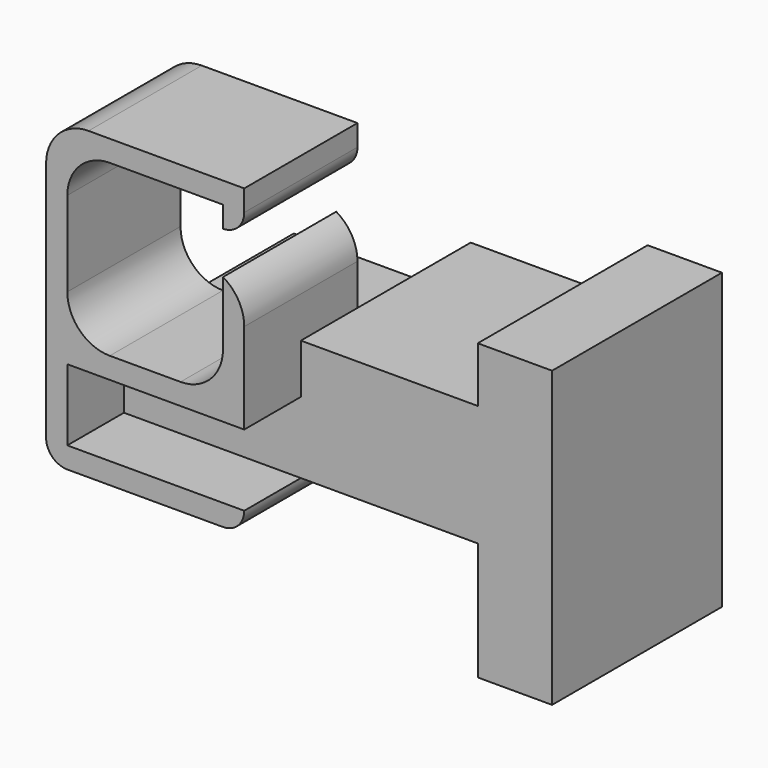
from build123d import *

# Parameters (mm, degrees)
F0_W          = 25
F0_H          = 7
F0_W_2        = 10.5
F0_H_2        = 10.1
F0_H_3        = 16.6735936701
F0_H_4        = 7.8
F1_DEPTH      = 15
F1_DEPTH_BACK = 15
F2_W          = 3
F2_H          = 3
F3_DEPTH      = 10
F3_DEPTH_BACK = 10
F4_T1_DEPTH   = 20
F4_T3_DEPTH   = 20
F4_T5_DEPTH   = 20
F4_T7_DEPTH   = 50
F4_T9_DEPTH   = 45.9807621135
F5_R          = 2.99999


# Not quite as in the source:
# - a fillet or chamfer that OpenCascade refuses, or shapes differently, is made with other operations: its cross-section is extruded or revolved along the edge and cut away or added
# - a fillet or chamfer is up to 0.001 mm smaller than in the source, because OpenCascade refuses the exact size
# - a feature names something its author has since deleted; it is built from what else it names


with BuildPart() as f1:
    # F0 (on Front) → F1 (new body, two sides)
    with BuildSketch(Plane.XZ) as f1_sk:
        Polygon((-5.5, 5.1), (-30.5, 5.1), (-30.5, -5), (19.5, -5), (19.5, 5.1), align=None)
        with Locations((7, 8.6)):
            Rectangle(F0_W, F0_H)
        with Locations((24.75, 8.6)):
            Rectangle(F0_W_2, F0_H)
        with Locations((24.75, 0.05)):
            Rectangle(F0_W_2, F0_H_2)
        with Locations((24.75, -13.3367968351)):
            Rectangle(F0_W_2, F0_H_3)
        with Locations((24.75, 16)):
            Rectangle(F0_W_2, F0_H_4)
    extrude(amount=F1_DEPTH)
    extrude(f1_sk.sketch, amount=-F1_DEPTH_BACK)


with BuildPart() as f3:
    # F2 (on face) → F3 (new body, two sides)
    with BuildSketch(Plane.XZ.offset(15)) as f3_sk:
        Polygon((-30.5, -5), (-30.5, 5.1), (-5.5, 5.1), (-5.5, 12.1), (-5.5, 23.1), (-8.5, 23.1), (-8.5, 15.1), (-8.5, 8.1), (-30.5, 8.1), (-30.5, 32.1), (-8.5, 32.1), (-5.5, 32.1), (-5.5, 35.1), (-33.5, 35.1), (-33.5, 8.1), (-33.5, -5), (-33.5, -8), (-5.5, -8), (-5.5, -5), align=None)
        with Locations((-7, 30.6)):
            Rectangle(F2_W, F2_H)
    extrude(amount=F3_DEPTH)
    extrude(f3_sk.sketch, amount=-F3_DEPTH_BACK)

    # F4: fillet of radius 6 on 5 edges, made by hand

    # F4_s2 → F4_t1 (join)
    with BuildSketch(Plane.XZ.offset(5)):
        with BuildLine():
            ThreePointArc((-24.5, 32.1), (-28.7426406871, 30.3426406871), (-30.5, 26.1))
            Line((-30.5, 26.1), (-30.5, 32.1))
            Line((-30.5, 32.1), (-24.5, 32.1))
        make_face()
    extrude(amount=F4_T1_DEPTH)

    # F4_s4 → F4_t3 (join)
    with BuildSketch(Plane.XZ.offset(5)):
        with BuildLine():
            ThreePointArc((-24.5, 8.1), (-28.7426406871, 9.8573593129), (-30.5, 14.1))
            Line((-30.5, 14.1), (-30.5, 8.1))
            Line((-30.5, 8.1), (-24.5, 8.1))
        make_face()
    extrude(amount=F4_T3_DEPTH)

    # F4_s6 → F4_t5 (join)
    with BuildSketch(Plane.XZ.offset(5)):
        with BuildLine():
            ThreePointArc((-8.5, 14.1), (-10.2573593129, 9.8573593129), (-14.5, 8.1))
            Line((-14.5, 8.1), (-8.5, 8.1))
            Line((-8.5, 8.1), (-8.5, 14.1))
        make_face()
    extrude(amount=F4_T5_DEPTH)

    # F4_s8 → F4_t7 (cut)
    with BuildSketch(Plane.XZ.offset(-10)):
        with BuildLine():
            ThreePointArc((-27.5, 35.1), (-31.7426406871, 33.3426406871), (-33.5, 29.1))
            Line((-33.5, 29.1), (-33.5, 35.1))
            Line((-33.5, 35.1), (-27.5, 35.1))
        make_face()
    extrude(amount=F4_T7_DEPTH, mode=Mode.SUBTRACT)

    # F4_s10 → F4_t9 (cut)
    with BuildSketch(Plane.XZ.offset(-7.9903810568)):
        with BuildLine():
            ThreePointArc((-8.5, 23.1), (-6.3038475773, 20.9038475773), (-5.5, 17.9038475773))
            Line((-5.5, 17.9038475773), (-5.5, 23.1))
            Line((-5.5, 23.1), (-8.5, 23.1))
        make_face()
    extrude(amount=F4_T9_DEPTH, mode=Mode.SUBTRACT)

    # F5 (radius 3 in the source; OpenCascade refuses exactly that, so slightly less here)
    f5_edges = [f3.edges().sort_by_distance(p)[0] for p in [
        (-33.5, -15, -8),
        (-5.5, -15, 29.1),
        (-5.5, -15, -8),
    ]]
    fillet(f5_edges, radius=F5_R)


solid = Compound([f1.part, f3.part])
